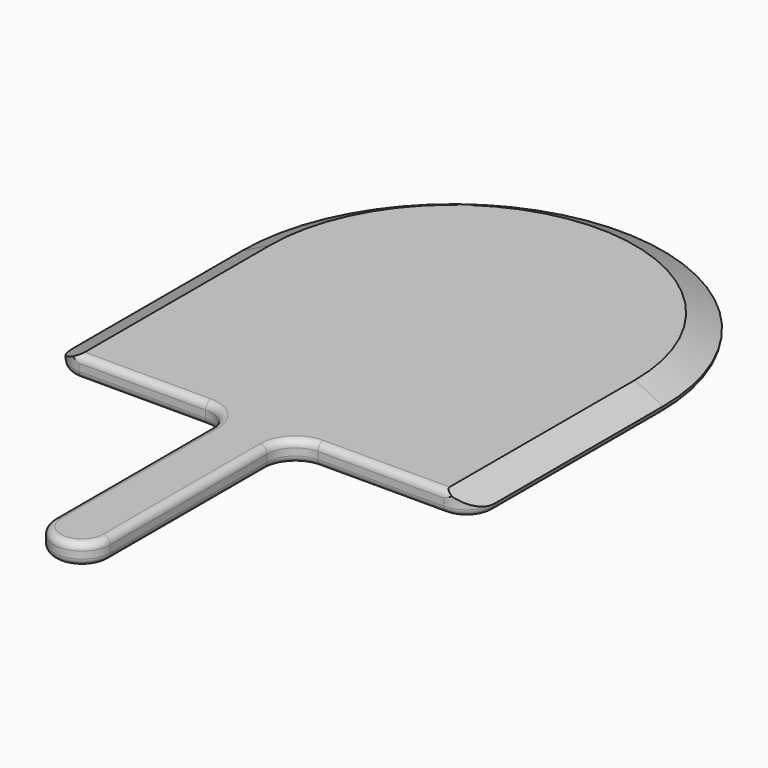
from build123d import *

# Parameters (mm, degrees)
F1_DEPTH    = 19.05
F2_T1_DEPTH = 256.2816533942
F2_T4_ANGLE = 180
F3_R        = 6.35
F4_R        = 6.34999


# Not quite as in the source:
# - a fillet or chamfer that OpenCascade refuses, or shapes differently, is made with other operations: its cross-section is extruded or revolved along the edge and cut away or added
# - a fillet or chamfer is up to 0.001 mm smaller than in the source, because OpenCascade refuses the exact size


with BuildPart() as f1:
    # F0 (on Top) → F1 (new body)
    with BuildSketch(Plane.XY):
        with BuildLine():
            Line((190.5, -190.5), (190.5, 0))
            ThreePointArc((190.5, 0), (0, 190.5), (-190.5, 0))
            Line((-190.5, 0), (-190.5, -190.5))
            ThreePointArc((-190.5, -190.5), (-183.0605122421, -208.4605122421), (-165.1, -215.9))
            Line((-165.1, -215.9), (-50.8, -215.9))
            ThreePointArc((-50.8, -215.9), (-32.8394877579, -223.3394877579), (-25.4, -241.3))
            Line((-25.4, -241.3), (-25.4, -419.1))
            ThreePointArc((-25.4, -419.1), (0, -444.5), (25.4, -419.1))
            Line((25.4, -419.1), (25.4, -241.3))
            ThreePointArc((25.4, -241.3), (32.8394877579, -223.3394877579), (50.8, -215.9))
            Line((50.8, -215.9), (165.1, -215.9))
            ThreePointArc((165.1, -215.9), (183.0605122421, -208.4605122421), (190.5, -190.5))
        make_face()
    extrude(amount=F1_DEPTH)

    # F2: chamfer of 12.7 x 25.4 on 3 edges, made by hand

    # F2_s2 → F2_t1 (cut)
    with BuildSketch(Plane.XZ):
        Polygon((-190.5, 6.35), (-165.1, 19.05), (-190.5, 19.05), align=None)
        Polygon((190.5, 6.35), (165.1, 19.05), (190.5, 19.05), align=None)
    extrude(amount=F2_T1_DEPTH, mode=Mode.SUBTRACT)

    # F2_s3 → F2_t4 (revolve, cut)
    with BuildSketch(Plane.XZ):
        Polygon((190.5, 6.35), (165.1, 19.05), (190.5, 19.05), align=None)
    revolve(axis=Axis((0, 0, 19.05), (0, 0, 1)), revolution_arc=F2_T4_ANGLE, mode=Mode.SUBTRACT)

    # F3
    f3_edges = [f1.edges().sort_by_distance(p)[0] for p in [
        (0, -444.5, 19.05),
    ]]
    fillet(f3_edges, radius=F3_R)

    # F4 (radius 6.35 in the source; OpenCascade refuses exactly that, so slightly less here)
    f4_edges = [f1.edges().sort_by_distance(p)[0] for p in [
        (25.4, -330.2, 0),
        (32.839488, -223.339488, 0),
        (107.95, -215.9, 0),
        (183.060512, -208.460512, 0),
        (190.5, -95.25, 0),
        (0, 190.5, 0),
        (-190.5, -95.25, 0),
        (-183.060512, -208.460512, 0),
        (-107.95, -215.9, 0),
        (-32.839488, -223.339488, 0),
        (-25.4, -330.2, 0),
        (0, -444.5, 0),
    ]]
    fillet(f4_edges, radius=F4_R)


solid = f1.part
